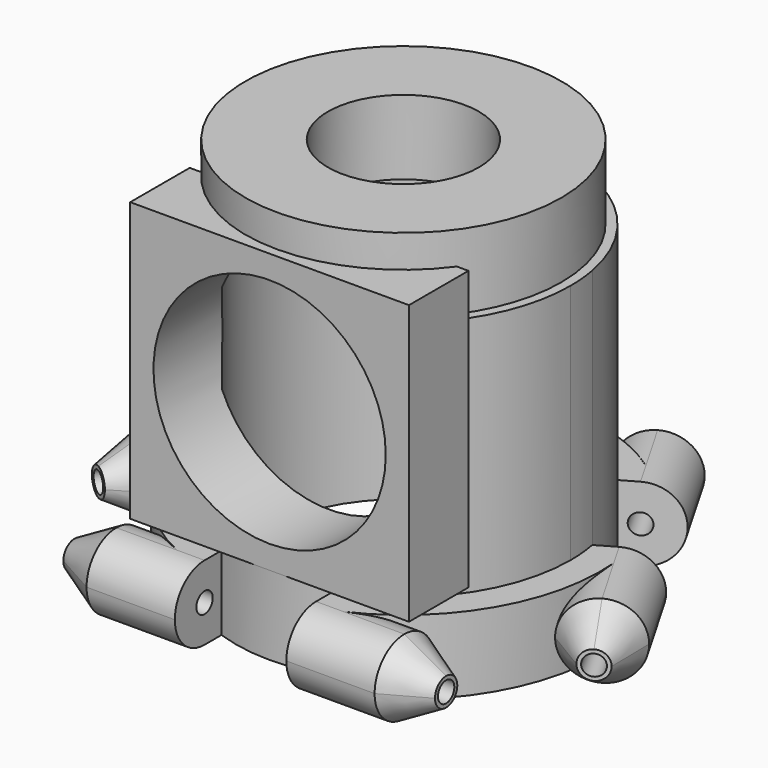
from build123d import *

# Parameters (mm, degrees)
F0_R         = 15.25
F1_DEPTH     = 8
F2_R         = 3.99999
F3_T1_DEPTH  = 2e-05
F3_T3_DEPTH  = 2e-05
F3_T5_DEPTH  = 2e-05
F3_T7_DEPTH  = 2e-05
F3_T9_DEPTH  = 2e-05
F3_T11_DEPTH = 2e-05
F3_T14_ANGLE = 90
F3_T16_ANGLE = 90
F3_T18_ANGLE = 90
F3_T20_ANGLE = 90
F3_T22_ANGLE = 90
F3_T24_ANGLE = 90
F3_T26_ANGLE = 90
F3_T28_ANGLE = 90
F3_T30_ANGLE = 90
F3_T32_ANGLE = 90
F3_T34_ANGLE = 90
F3_T36_ANGLE = 90
F3_T38_ANGLE = 90
F3_T40_ANGLE = 90
F3_T42_ANGLE = 90
F3_T44_ANGLE = 90
F3_T46_ANGLE = 90
F3_T48_ANGLE = 90
F3_T50_ANGLE = 90
F3_T52_ANGLE = 90
F3_T54_ANGLE = 90
F3_T56_ANGLE = 90
F3_T58_ANGLE = 90
F3_T60_ANGLE = 90
F4_R         = 1.1
F5_DEPTH     = 41
F6_R         = 1.1
F7_DEPTH     = 41
F8_R         = 1.1
F9_DEPTH     = 41
F10_R        = 15.25
F11_DEPTH    = 26
F12_R        = 17
F12_R_2      = 8.125
F13_DEPTH    = 8
F15_START    = 10
F14_W        = 30
F14_H        = 30
F15_DEPTH    = 8
F16_R        = 12.5
F17_DEPTH    = 10


# Not quite as in the source:
# - a fillet or chamfer that OpenCascade refuses, or shapes differently, is made with other operations: its cross-section is extruded or revolved along the edge and cut away or added
# - a fillet or chamfer is up to 0.001 mm smaller than in the source, because OpenCascade refuses the exact size


with BuildPart() as f1:
    # F0 (on Top) → F1 (new body)
    with BuildSketch(Plane.XY):
        with BuildLine():
            Line((-6, -23.25), (-6, -16.9705627485))
            ThreePointArc((-6, -16.9705627485), (0, -18), (6, -16.9705627485))
            Line((6, -16.9705627485), (6, -23.25))
            Line((6, -23.25), (20, -23.25))
            Line((20, -23.25), (20, -15.25))
            Line((20, -15.25), (14.7811478747, -15.25))
            ThreePointArc((14.7811478747, -15.25), (18.3924468792, -10.6188841567), (20.5974613451, -5.1758495566))
            Line((20.5974613451, -5.1758495566), (23.2068874077, -9.6955080757))
            Line((23.2068874077, -9.6955080757), (30.135090638, -5.6955080757))
            Line((30.135090638, -5.6955080757), (23.135090638, 6.4288475773))
            Line((23.135090638, 6.4288475773), (17.6969384567, 3.2891289515))
            ThreePointArc((17.6969384567, 3.2891289515), (15.5884572681, 9), (11.6969384567, 13.6814337969))
            Line((11.6969384567, 13.6814337969), (17.135090638, 16.8211524227))
            Line((17.135090638, 16.8211524227), (10.135090638, 28.9455080757))
            Line((10.135090638, 28.9455080757), (3.2068874077, 24.9455080757))
            Line((3.2068874077, 24.9455080757), (5.8163134704, 20.4258495566))
            ThreePointArc((5.8163134704, 20.4258495566), (0, 21.2377683135), (-5.8163134704, 20.4258495566))
            Line((-5.8163134704, 20.4258495566), (-3.2068874077, 24.9455080757))
            Line((-3.2068874077, 24.9455080757), (-10.135090638, 28.9455080757))
            Line((-10.135090638, 28.9455080757), (-17.135090638, 16.8211524227))
            Line((-17.135090638, 16.8211524227), (-11.6969384567, 13.6814337969))
            ThreePointArc((-11.6969384567, 13.6814337969), (-15.5884572681, 9), (-17.6969384567, 3.2891289515))
            Line((-17.6969384567, 3.2891289515), (-23.135090638, 6.4288475773))
            Line((-23.135090638, 6.4288475773), (-30.135090638, -5.6955080757))
            Line((-30.135090638, -5.6955080757), (-23.2068874077, -9.6955080757))
            Line((-23.2068874077, -9.6955080757), (-20.5974613451, -5.1758495566))
            ThreePointArc((-20.5974613451, -5.1758495566), (-18.3924468792, -10.6188841567), (-14.7811478747, -15.25))
            Line((-14.7811478747, -15.25), (-20, -15.25))
            Line((-20, -15.25), (-20, -23.25))
            Line((-20, -23.25), (-6, -23.25))
        make_face()
        Circle(F0_R, mode=Mode.SUBTRACT)
    extrude(amount=F1_DEPTH)

    # F2 (radius 4 in the source; OpenCascade refuses exactly that, so slightly less here)
    f2_edges = [f1.edges().sort_by_distance(p)[0] for p in [
        (13.635091, 22.88333, 8),
        (26.635091, 0.36667, 8),
        (13, -23.25, 8),
        (-13, -23.25, 8),
        (-26.635091, 0.36667, 8),
        (-13.635091, 22.88333, 8),
        (-4.5116, 22.685679, 8),
        (4.5116, 22.685679, 8),
        (21.902174, -7.435679, 8),
        (17.390574, -15.25, 8),
        (-17.390574, -15.25, 8),
        (-21.902174, -7.435679, 8),
        (-13.635091, 22.88333, 0),
        (-26.635091, 0.36667, 0),
        (-13, -23.25, 0),
        (13, -23.25, 0),
        (26.635091, 0.36667, 0),
        (13.635091, 22.88333, 0),
        (4.5116, 22.685679, 0),
        (-4.5116, 22.685679, 0),
        (-21.902174, -7.435679, 0),
        (-17.390574, -15.25, 0),
        (17.390574, -15.25, 0),
        (21.902174, -7.435679, 0),
    ]]
    fillet(f2_edges, radius=F2_R)

    # F3: chamfer of 2.5 x 4.5 on 48 edges, made by hand

    # F3_s2 → F3_t1 (cut)
    with BuildSketch(Plane.XY.offset(3.99999)):
        Polygon((-20.9568874077, -5.7983937587), (-25.3719509172, -8.4455080757), (-23.2068874077, -9.6955080757), align=None)
        Polygon((-15.5, -15.25), (-20, -17.75), (-20, -15.25), align=None)
        Polygon((-27.9700271285, -6.9455080757), (-27.885090638, -1.7983937587), (-30.135090638, -5.6955080757), align=None)
        Polygon((-20, -20.75), (-15.5, -23.25), (-20, -23.25), align=None)
        Polygon((20, -20.75), (15.5, -23.25), (20, -23.25), align=None)
        Polygon((20, -17.75), (15.5, -15.25), (20, -15.25), align=None)
        Polygon((-5.3719509172, 26.1955080757), (-5.4568874077, 21.0483937587), (-3.2068874077, 24.9455080757), align=None)
        Polygon((-7.9700271285, 27.6955080757), (-12.385090638, 25.0483937587), (-10.135090638, 28.9455080757), align=None)
        Polygon((25.3719509172, -8.4455080757), (20.9568874077, -5.7983937587), (23.2068874077, -9.6955080757), align=None)
        Polygon((27.9700271285, -6.9455080757), (27.885090638, -1.7983937587), (30.135090638, -5.6955080757), align=None)
        Polygon((7.9700271285, 27.6955080757), (12.385090638, 25.0483937587), (10.135090638, 28.9455080757), align=None)
        Polygon((5.3719509172, 26.1955080757), (5.4568874077, 21.0483937587), (3.2068874077, 24.9455080757), align=None)
    extrude(amount=F3_T1_DEPTH, mode=Mode.SUBTRACT)

    # F3_s4 → F3_t3 (cut)
    with BuildSketch(Plane.XZ.offset(19.24999)):
        Polygon((-15.5, 0), (-20, 2.5), (-20, 0), align=None)
        Polygon((15.5, 0), (20, 2.5), (20, 0), align=None)
        Polygon((-15.5, 8), (-20, 5.5), (-20, 8), align=None)
        Polygon((15.5, 8), (20, 5.5), (20, 8), align=None)
    extrude(amount=F3_T3_DEPTH, mode=Mode.SUBTRACT)

    # F3_s6 → F3_t5 (cut)
    with BuildSketch(Plane(origin=(-16.6709976831, 9.625005, 0), x_dir=(0, 0, 1), z_dir=(0.8660254038, -0.5, 0))):
        Polygon((0, 15.5), (2.5, 20), (0, 20), align=None)
        Polygon((8, 15.5), (5.5, 20), (8, 20), align=None)
    extrude(amount=F3_T5_DEPTH, mode=Mode.SUBTRACT)

    # F3_s8 → F3_t7 (cut)
    with BuildSketch(Plane(origin=(-16.6709803626, 9.624995, 0), x_dir=(0, 0, 1), z_dir=(-0.8660254038, 0.5, 0))):
        Polygon((0, 15.5), (2.5, 20), (0, 20), align=None)
        Polygon((8, 15.5), (5.5, 20), (8, 20), align=None)
    extrude(amount=F3_T7_DEPTH, mode=Mode.SUBTRACT)

    # F3_s10 → F3_t9 (cut)
    with BuildSketch(Plane(origin=(16.6709803626, 9.624995, 0), x_dir=(0, 0, 1), z_dir=(0.8660254038, 0.5, 0))):
        Polygon((0, 15.5), (2.5, 20), (0, 20), align=None)
        Polygon((8, 15.5), (5.5, 20), (8, 20), align=None)
    extrude(amount=F3_T9_DEPTH, mode=Mode.SUBTRACT)

    # F3_s12 → F3_t11 (cut)
    with BuildSketch(Plane(origin=(16.6709976831, 9.625005, 0), x_dir=(0, 0, 1), z_dir=(-0.8660254038, -0.5, 0))):
        Polygon((0, 15.5), (2.5, 20), (0, 20), align=None)
        Polygon((8, 15.5), (5.5, 20), (8, 20), align=None)
    extrude(amount=F3_T11_DEPTH, mode=Mode.SUBTRACT)

    # F3_s13 → F3_t14 (revolve, cut)
    with BuildSketch(Plane.XY.offset(3.99999)):
        Polygon((-27.9700271285, -6.9455080757), (-27.885090638, -1.7983937587), (-30.135090638, -5.6955080757), align=None)
    revolve(axis=Axis((-26.6709976831, -7.6955030757, 3.99999), (-0.5, -0.8660254038, 0)), revolution_arc=F3_T14_ANGLE, mode=Mode.SUBTRACT)

    # F3_s15 → F3_t16 (revolve, cut)
    with BuildSketch(Plane.XY.offset(3.99999)):
        Polygon((12.385090638, 25.0483937587), (7.9700271285, 27.6955080757), (10.135090638, 28.9455080757), align=None)
    revolve(axis=Axis((6.6709976831, 26.9455130757, 3.99999), (-0.5, 0.8660254038, 0)), revolution_arc=F3_T16_ANGLE, mode=Mode.SUBTRACT)

    # F3_s17 → F3_t18 (revolve, cut)
    with BuildSketch(Plane.XY.offset(3.99999)):
        Polygon((20.9568874077, -5.7983937587), (25.3719509172, -8.4455080757), (23.2068874077, -9.6955080757), align=None)
    revolve(axis=Axis((26.6709803626, -7.6955130757, 3.99999), (0.5, -0.8660254038, 0)), revolution_arc=F3_T18_ANGLE, mode=Mode.SUBTRACT)

    # F3_s19 → F3_t20 (revolve, cut)
    with BuildSketch(Plane.XY.offset(3.99999)):
        Polygon((15.5, -23.25), (20, -20.75), (20, -23.25), align=None)
    revolve(axis=Axis((20, -19.25001, 3.99999), (1, 0, 0)), revolution_arc=F3_T20_ANGLE, mode=Mode.SUBTRACT)

    # F3_s21 → F3_t22 (revolve, cut)
    with BuildSketch(Plane.XY.offset(3.99999)):
        Polygon((-15.5, -15.25), (-20, -17.75), (-20, -15.25), align=None)
    revolve(axis=Axis((-20, -19.24999, 3.99999), (-1, 0, 0)), revolution_arc=F3_T22_ANGLE, mode=Mode.SUBTRACT)

    # F3_s23 → F3_t24 (revolve, cut)
    with BuildSketch(Plane.XY.offset(3.99999)):
        Polygon((-5.3719509172, 26.1955080757), (-5.4568874077, 21.0483937587), (-3.2068874077, 24.9455080757), align=None)
    revolve(axis=Axis((-6.6709803626, 26.9455030757, 3.99999), (0.5, 0.8660254038, 0)), revolution_arc=F3_T24_ANGLE, mode=Mode.SUBTRACT)

    # F3_s25 → F3_t26 (revolve, cut)
    with BuildSketch(Plane.XY.offset(3.99999)):
        Polygon((-20.9568874077, -5.7983937587), (-25.3719509172, -8.4455080757), (-23.2068874077, -9.6955080757), align=None)
    revolve(axis=Axis((-26.6709803626, -7.6955130757, 3.99999), (0.5, 0.8660254038, 0)), revolution_arc=F3_T26_ANGLE, mode=Mode.SUBTRACT)

    # F3_s27 → F3_t28 (revolve, cut)
    with BuildSketch(Plane.XY.offset(4.00001)):
        Polygon((-20.9568874077, -5.7983937587), (-25.3719509172, -8.4455080757), (-23.2068874077, -9.6955080757), align=None)
    revolve(axis=Axis((-26.6709803626, -7.6955130757, 4.00001), (-0.5, -0.8660254038, 0)), revolution_arc=F3_T28_ANGLE, mode=Mode.SUBTRACT)

    # F3_s29 → F3_t30 (revolve, cut)
    with BuildSketch(Plane.XY.offset(4.00001)):
        Polygon((-15.5, -15.25), (-20, -17.75), (-20, -15.25), align=None)
    revolve(axis=Axis((-20, -19.24999, 4.00001), (1, 0, 0)), revolution_arc=F3_T30_ANGLE, mode=Mode.SUBTRACT)

    # F3_s31 → F3_t32 (revolve, cut)
    with BuildSketch(Plane.XY.offset(4.00001)):
        Polygon((-27.9700271285, -6.9455080757), (-27.885090638, -1.7983937587), (-30.135090638, -5.6955080757), align=None)
    revolve(axis=Axis((-26.6709976831, -7.6955030757, 4.00001), (0.5, 0.8660254038, 0)), revolution_arc=F3_T32_ANGLE, mode=Mode.SUBTRACT)

    # F3_s33 → F3_t34 (revolve, cut)
    with BuildSketch(Plane.XY.offset(3.99999)):
        Polygon((-20, -20.75), (-15.5, -23.25), (-20, -23.25), align=None)
    revolve(axis=Axis((-20, -19.25001, 3.99999), (1, 0, 0)), revolution_arc=F3_T34_ANGLE, mode=Mode.SUBTRACT)

    # F3_s35 → F3_t36 (revolve, cut)
    with BuildSketch(Plane.XY.offset(4.00001)):
        Polygon((-20, -20.75), (-15.5, -23.25), (-20, -23.25), align=None)
    revolve(axis=Axis((-20, -19.25001, 4.00001), (-1, 0, 0)), revolution_arc=F3_T36_ANGLE, mode=Mode.SUBTRACT)

    # F3_s37 → F3_t38 (revolve, cut)
    with BuildSketch(Plane.XY.offset(4.00001)):
        Polygon((20, -20.75), (15.5, -23.25), (20, -23.25), align=None)
    revolve(axis=Axis((20, -19.25001, 4.00001), (-1, 0, 0)), revolution_arc=F3_T38_ANGLE, mode=Mode.SUBTRACT)

    # F3_s39 → F3_t40 (revolve, cut)
    with BuildSketch(Plane.XY.offset(3.99999)):
        Polygon((20, -17.75), (15.5, -15.25), (20, -15.25), align=None)
    revolve(axis=Axis((20, -19.24999, 3.99999), (-1, 0, 0)), revolution_arc=F3_T40_ANGLE, mode=Mode.SUBTRACT)

    # F3_s41 → F3_t42 (revolve, cut)
    with BuildSketch(Plane.XY.offset(4.00001)):
        Polygon((20, -17.75), (15.5, -15.25), (20, -15.25), align=None)
    revolve(axis=Axis((20, -19.24999, 4.00001), (1, 0, 0)), revolution_arc=F3_T42_ANGLE, mode=Mode.SUBTRACT)

    # F3_s43 → F3_t44 (revolve, cut)
    with BuildSketch(Plane.XY.offset(3.99999)):
        Polygon((-12.385090638, 25.0483937587), (-7.9700271285, 27.6955080757), (-10.135090638, 28.9455080757), align=None)
    revolve(axis=Axis((-6.6709976831, 26.9455130757, 3.99999), (-0.5, -0.8660254038, 0)), revolution_arc=F3_T44_ANGLE, mode=Mode.SUBTRACT)

    # F3_s45 → F3_t46 (revolve, cut)
    with BuildSketch(Plane.XY.offset(4.00001)):
        Polygon((-5.3719509172, 26.1955080757), (-5.4568874077, 21.0483937587), (-3.2068874077, 24.9455080757), align=None)
    revolve(axis=Axis((-6.6709803626, 26.9455030757, 4.00001), (-0.5, -0.8660254038, 0)), revolution_arc=F3_T46_ANGLE, mode=Mode.SUBTRACT)

    # F3_s47 → F3_t48 (revolve, cut)
    with BuildSketch(Plane.XY.offset(4.00001)):
        Polygon((-7.9700271285, 27.6955080757), (-12.385090638, 25.0483937587), (-10.135090638, 28.9455080757), align=None)
    revolve(axis=Axis((-6.6709976831, 26.9455130757, 4.00001), (0.5, 0.8660254038, 0)), revolution_arc=F3_T48_ANGLE, mode=Mode.SUBTRACT)

    # F3_s49 → F3_t50 (revolve, cut)
    with BuildSketch(Plane.XY.offset(4.00001)):
        Polygon((25.3719509172, -8.4455080757), (20.9568874077, -5.7983937587), (23.2068874077, -9.6955080757), align=None)
    revolve(axis=Axis((26.6709803626, -7.6955130757, 4.00001), (-0.5, 0.8660254038, 0)), revolution_arc=F3_T50_ANGLE, mode=Mode.SUBTRACT)

    # F3_s51 → F3_t52 (revolve, cut)
    with BuildSketch(Plane.XY.offset(3.99999)):
        Polygon((27.9700271285, -6.9455080757), (27.885090638, -1.7983937587), (30.135090638, -5.6955080757), align=None)
    revolve(axis=Axis((26.6709976831, -7.6955030757, 3.99999), (-0.5, 0.8660254038, 0)), revolution_arc=F3_T52_ANGLE, mode=Mode.SUBTRACT)

    # F3_s53 → F3_t54 (revolve, cut)
    with BuildSketch(Plane.XY.offset(4.00001)):
        Polygon((27.9700271285, -6.9455080757), (27.885090638, -1.7983937587), (30.135090638, -5.6955080757), align=None)
    revolve(axis=Axis((26.6709976831, -7.6955030757, 4.00001), (0.5, -0.8660254038, 0)), revolution_arc=F3_T54_ANGLE, mode=Mode.SUBTRACT)

    # F3_s55 → F3_t56 (revolve, cut)
    with BuildSketch(Plane.XY.offset(3.99999)):
        Polygon((5.4568874077, 21.0483937587), (5.3719509172, 26.1955080757), (3.2068874077, 24.9455080757), align=None)
    revolve(axis=Axis((6.6709803626, 26.9455030757, 3.99999), (0.5, -0.8660254038, 0)), revolution_arc=F3_T56_ANGLE, mode=Mode.SUBTRACT)

    # F3_s57 → F3_t58 (revolve, cut)
    with BuildSketch(Plane.XY.offset(4.00001)):
        Polygon((7.9700271285, 27.6955080757), (12.385090638, 25.0483937587), (10.135090638, 28.9455080757), align=None)
    revolve(axis=Axis((6.6709976831, 26.9455130757, 4.00001), (0.5, -0.8660254038, 0)), revolution_arc=F3_T58_ANGLE, mode=Mode.SUBTRACT)

    # F3_s59 → F3_t60 (revolve, cut)
    with BuildSketch(Plane.XY.offset(4.00001)):
        Polygon((5.3719509172, 26.1955080757), (5.4568874077, 21.0483937587), (3.2068874077, 24.9455080757), align=None)
    revolve(axis=Axis((6.6709803626, 26.9455030757, 4.00001), (-0.5, 0.8660254038, 0)), revolution_arc=F3_T60_ANGLE, mode=Mode.SUBTRACT)

    # F4 (on face) → F5 (cut)
    with BuildSketch(Plane(origin=(-10, -17.3205080757, 0), x_dir=(0.8660254038, -0.5, 0), z_dir=(-0.5, -0.8660254038, 0))):
        with Locations((-19.25, 4)):
            Circle(F4_R)
    extrude(amount=-F5_DEPTH, mode=Mode.SUBTRACT)

    # F6 (on face) → F7 (cut)
    with BuildSketch(Plane(origin=(-20, 0, 0), x_dir=(0, -1, 0), z_dir=(-1, 0, 0))):
        with Locations((19.25, 4)):
            Circle(F6_R)
    extrude(amount=-F7_DEPTH, mode=Mode.SUBTRACT)

    # F8 (on face) → F9 (cut)
    with BuildSketch(Plane(origin=(10, -17.3205080757, 0), x_dir=(0.8660254038, 0.5, 0), z_dir=(0.5, -0.8660254038, 0))):
        with Locations((19.25, 4)):
            Circle(F8_R)
    extrude(amount=-F9_DEPTH, mode=Mode.SUBTRACT)

    # F10 (on face) → F11 (join)
    with BuildSketch(Plane.XY.offset(8)):
        with BuildLine():
            ThreePointArc((6, -16.9705627485), (14.6969384567, -10.3923048454), (18, 0))
            ThreePointArc((18, 0), (17.9240744841, 1.6515307717), (17.6969384567, 3.2891289515))
            ThreePointArc((17.6969384567, 3.2891289515), (15.5884572681, 9), (11.6969384567, 13.6814337969))
            ThreePointArc((11.6969384567, 13.6814337969), (0, 18), (-11.6969384567, 13.6814337969))
            ThreePointArc((-11.6969384567, 13.6814337969), (-15.5884572681, 9), (-17.6969384567, 3.2891289515))
            ThreePointArc((-17.6969384567, 3.2891289515), (-15.5884572681, -9), (-6, -16.9705627485))
            ThreePointArc((-6, -16.9705627485), (0, -18), (6, -16.9705627485))
        make_face()
        Circle(F10_R, mode=Mode.SUBTRACT)
    extrude(amount=F11_DEPTH)

    # F12 (on face) → F13 (join)
    with BuildSketch(Plane.XY.offset(34)):
        Circle(F12_R)
        Circle(F12_R_2, mode=Mode.SUBTRACT)
    extrude(amount=F13_DEPTH)

    # F14 (on Front) → F15 (join)
    with BuildSketch(Plane.XZ.offset(F15_START)):
        with Locations((0, 23.5)):
            Rectangle(F14_W, F14_H)
    extrude(amount=F15_DEPTH)

    # F16 (on face) → F17 (cut)
    with BuildSketch(Plane.XZ.offset(18)):
        with Locations((0, 23.5)):
            Circle(F16_R)
    extrude(amount=-F17_DEPTH, mode=Mode.SUBTRACT)


solid = f1.part
